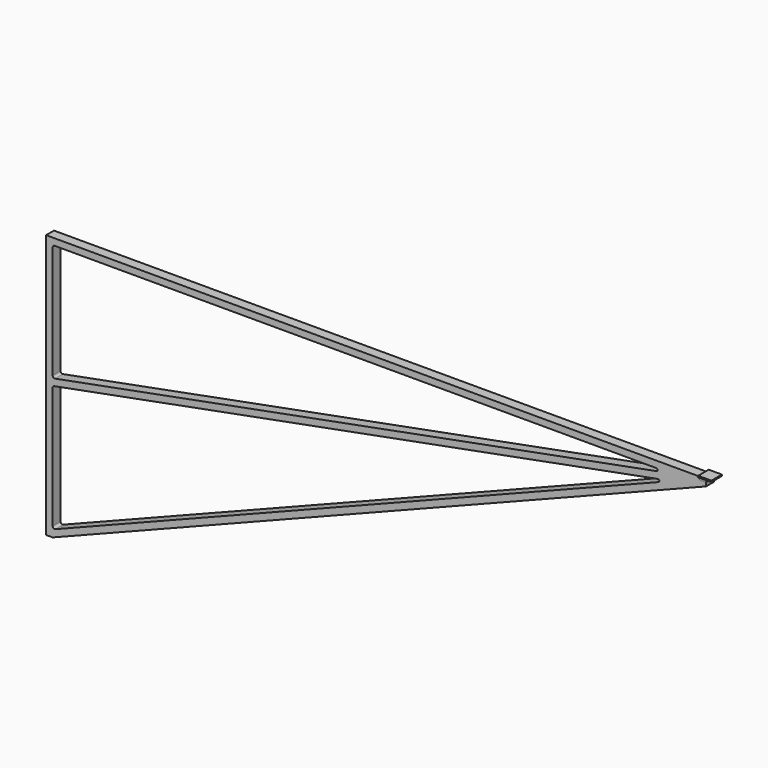
from build123d import *

# Parameters (mm, degrees)
F1_DEPTH     = 7.5
F2_R         = 1.5
F3_R         = 1.5
F4_F1_R      = 1
F4_F2_R      = 1
F5_W         = 10
F5_H         = 10
F6_DEPTH     = 1
F7_T1_DEPTH  = 5
F7_T3_DEPTH  = 7.5
F7_T9_DEPTH  = 11.0917464655
F7_T14_DEPTH = 15
F7_T22_DEPTH = 15
F7_T27_DEPTH = 11.0917464655


# Not quite as in the source:
# - a fillet or chamfer that OpenCascade refuses, or shapes differently, is made with other operations: its cross-section is extruded or revolved along the edge and cut away or added


with BuildPart() as f1:
    # F0 (on Front) → F1 (new body)
    with BuildSketch(Plane.XZ):
        Polygon((0, 0), (0, 5), (-14.5909318536, 5), (-495, 5), (-500, 5), (-500, 0), (-500, -195), (-495, -195), (-408.1860127931, -160.8005504943), align=None)
        Polygon((-26.1103633187, -4.911916504), (-410.018635385, -156.1485085302), (-495, -189.6260158027), (-495, -142.4539996661), (-495, -95.2819835295), (-495, -93.9333955313), (-494.06737982, -93.7563320577), align=None, mode=Mode.SUBTRACT)
        Polygon((-495, 0), (-27.044750547, 0), (-495, -88.8440800691), (-495, -44.4220400346), align=None, mode=Mode.SUBTRACT)
    extrude(amount=F1_DEPTH)

    # F2
    f2_edges = [f1.edges().sort_by_distance(p)[0] for p in [
        (-495, -3.75, -88.84408),
    ]]
    fillet(f2_edges, radius=F2_R)

    # F3
    f3_edges = [f1.edges().sort_by_distance(p)[0] for p in [
        (-495, -3.75, -93.933396),
        (-495, -3.75, 0),
        (-495, -3.75, -189.626016),
    ]]
    fillet(f3_edges, radius=F3_R)

    # F4: fillet of radius 1 on 2 edges, made by hand

    # F4_f1
    f4_f1_edges = [f1.edges().sort_by_distance(p)[0] for p in [
        (-27.044750547, -3.75, 0),
    ]]
    fillet(f4_f1_edges, radius=F4_F1_R)

    # F4_f2
    f4_f2_edges = [f1.edges().sort_by_distance(p)[0] for p in [
        (-26.1103633187, -3.75, -4.911916504),
    ]]
    fillet(f4_f2_edges, radius=F4_F2_R)

    # F5 (on face) → F6 (join)
    with BuildSketch(Plane.XY.offset(5)):
        with Locations((0, -3.75)):
            Rectangle(F5_W, F5_H)
    extrude(amount=F6_DEPTH)

    # F7: fillet of radius 3 on 3 edges, made by hand

    # F7_s2 → F7_t1 (join)
    with BuildSketch(Plane.YZ.offset(-5)):
        with BuildLine():
            ThreePointArc((-7.5, 2.5633014138), (-7.830730437, 3.9326078076), (-8.75, 5))
            Line((-8.75, 5), (-7.5, 5))
            Line((-7.5, 5), (-7.5, 2.5633014138))
        make_face()
        with BuildLine():
            ThreePointArc((1.25, 5), (0.330730437, 3.9326078076), (0, 2.5633014138))
            Line((0, 2.5633014138), (0, 5))
            Line((0, 5), (1.25, 5))
        make_face()
    extrude(amount=F7_T1_DEPTH)

    # F7_s4 → F7_t3 (join)
    with BuildSketch(Plane.XZ):
        with BuildLine():
            ThreePointArc((0, 2), (0.8786796564, 4.1213203436), (3, 5))
            Line((3, 5), (0, 5))
            Line((0, 5), (0, 2))
        make_face()
    extrude(amount=F7_T3_DEPTH)


with BuildPart() as f7_tool7:
    # F7_s8 → F7_t9 (new body)
    with BuildSketch(Plane.YZ.offset(-5)):
        with BuildLine():
            ThreePointArc((-7.5, 2.5633014138), (-7.830730437, 3.9326078076), (-8.75, 5))
            Line((-8.75, 5), (-7.5, 5))
            Line((-7.5, 5), (-7.5, 2.5633014138))
        make_face()
    extrude(amount=F7_T9_DEPTH)

    split(bisect_by=Plane.YZ, keep=Keep.TOP)

    split(bisect_by=Plane.YZ.offset(5), keep=Keep.BOTTOM)


with BuildPart() as f7_tool12:
    # F7_s13 → F7_t14 (new body)
    with BuildSketch(Plane.XZ):
        with BuildLine():
            ThreePointArc((0, 2), (0.8786796564, 4.1213203436), (3, 5))
            Line((3, 5), (0, 5))
            Line((0, 5), (0, 2))
        make_face()
    extrude(amount=F7_T14_DEPTH)

    split(bisect_by=Plane.XZ.offset(7.5), keep=Keep.TOP)

    split(bisect_by=Plane.XZ.offset(8.75), keep=Keep.BOTTOM)


with BuildPart() as f7_tool7_1:
    add(f7_tool7.part)

    # F7_t17: intersect F7_tool12
    add(f7_tool12.part, mode=Mode.INTERSECT)


with BuildPart() as f1_1:
    add(f1.part)

    # F7_t5: union F7_tool7
    add(f7_tool7_1.part)


with BuildPart() as f7_tool20:
    # F7_s21 → F7_t22 (new body)
    with BuildSketch(Plane.XZ.offset(-7.5)):
        with BuildLine():
            ThreePointArc((0, 2), (0.8786796564, 4.1213203436), (3, 5))
            Line((3, 5), (0, 5))
            Line((0, 5), (0, 2))
        make_face()
    extrude(amount=F7_T22_DEPTH)

    split(bisect_by=Plane.XZ, keep=Keep.BOTTOM)

    split(bisect_by=Plane.XZ.offset(-1.25), keep=Keep.TOP)


with BuildPart() as f7_tool25:
    # F7_s26 → F7_t27 (new body)
    with BuildSketch(Plane.YZ.offset(6.0917464655)):
        with BuildLine():
            ThreePointArc((1.25, 5), (0.330730437, 3.9326078076), (0, 2.5633014138))
            Line((0, 2.5633014138), (0, 5))
            Line((0, 5), (1.25, 5))
        make_face()
    extrude(amount=-F7_T27_DEPTH)

    split(bisect_by=Plane.YZ, keep=Keep.TOP)

    split(bisect_by=Plane.YZ.offset(5), keep=Keep.BOTTOM)


with BuildPart() as f7_tool20_1:
    add(f7_tool20.part)

    # F7_t30: intersect F7_tool25
    add(f7_tool25.part, mode=Mode.INTERSECT)


with BuildPart() as f1_2:
    add(f1_1.part)

    # F7_t18: union F7_tool20
    add(f7_tool20_1.part)


solid = f1_2.part
